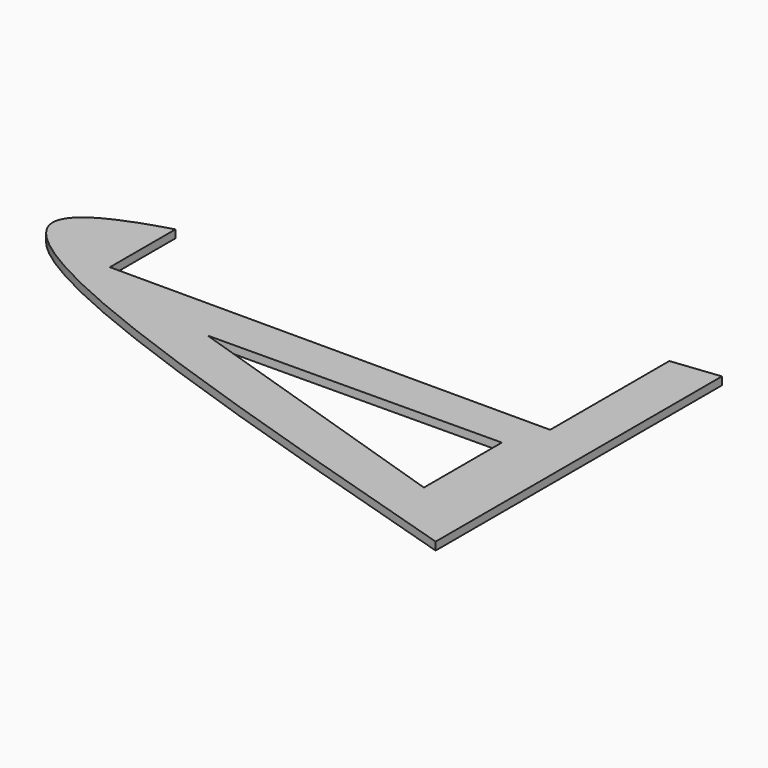
from build123d import *

# Parameters (mm, degrees)
F1_DEPTH = 0.6274920888


with BuildPart() as f1:
    # F0 (on Top) → F1 (new body)
    with BuildSketch(Plane.XY):
        with BuildLine():
            add(Edge.make_bspline(
                [(0, -18.7230408192), (-22.8005940455, -11.7347187551), (-52.7318931928, -2.5608557428), (-42.6186198614, 2.7495160437), (-38.6679108208, 3.8659247252)],
                knots=[0, 0, 0, 0, 0.5071475473, 0.6657537861, 0.6657537861, 0.6657537861, 0.6657537861], degree=3))
            Line((0, -18.7230408192), (0, -2.6170264397))
            Line((0, -2.6170264397), (0, 9.6031874418))
            add(Edge.make_bspline(
                [(-3.8220100603, 9.1760117782), (-2.5507177683, 9.3186652316), (-1.275358836, 9.4609263335), (0, 9.6031874418)],
                knots=[0.9719015733, 0.9719015733, 0.9719015733, 0.9719015733, 1, 1, 1, 1], degree=3))
            Line((-3.8220100603, 9.1760117782), (-3.8220100603, -2.6170264397))
            Line((-3.8220100603, -2.6170264397), (-38.6679108208, -2.6170264397))
            Line((-38.6679108208, -2.6170264397), (-38.6679108208, 3.8659247252))
        make_face()
        Polygon((-5.0867283717, -13.5254897177), (-28.2443165779, -5.9904903173), (-5.0867283717, -5.8171749115), align=None, mode=Mode.SUBTRACT)
    extrude(amount=F1_DEPTH)


solid = f1.part
